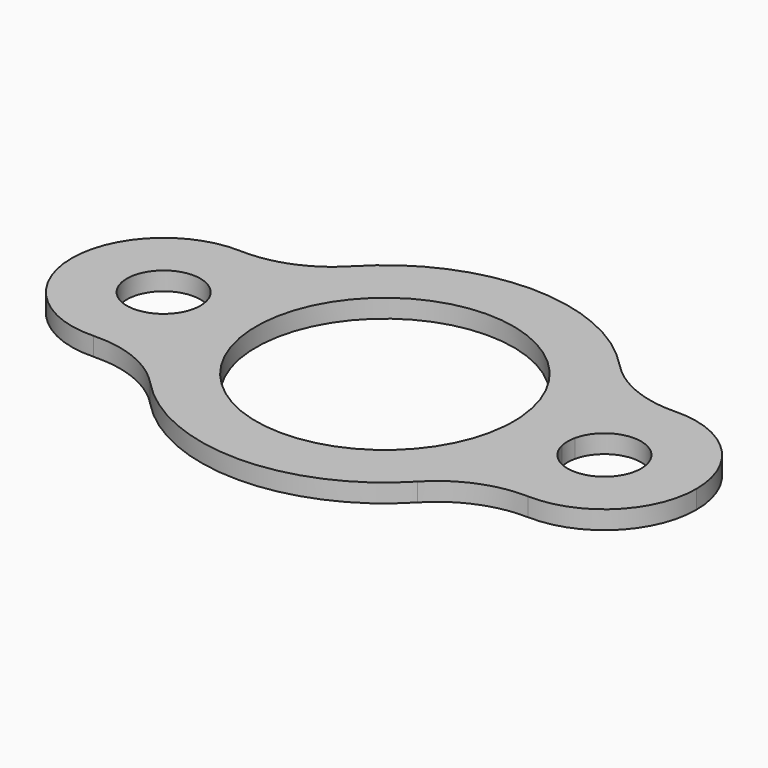
from build123d import *

# Parameters (mm, degrees)
F0_R     = 12.7
F1_DEPTH = 6.35
F2_R     = 38.1


# Not quite as in the source:
# - a length typed as a fraction of an inch, garbled in the dataset ("3 / 203.2 mm" for 3/8 in), is restored


with BuildPart() as f1:
    # F0 (on Top) → F1 (new body)
    with BuildSketch(Plane.XY):
        with BuildLine():
            ThreePointArc((44.2896283804, 3.7724419046), (44.4098889973, 1.8879245867), (44.45, 0))
            ThreePointArc((44.45, 0), (44.4098889973, -1.8879245867), (44.2896283804, -3.7724419046))
            ThreePointArc((44.2896283804, -3.7724419046), (48.6524538165, -16.4400117074), (57.8519523886, -26.1801757984))
            ThreePointArc((57.8519523886, -26.1801757983), (61.7568132692, -14.7765359551), (63.4364387448, -2.8404646402))
            ThreePointArc((63.4364387448, -2.8404646402), (63.1147165179, 0), (63.4364387448, 2.8404646402))
            ThreePointArc((63.4364387448, 2.8404646402), (61.7568132692, 14.7765359551), (57.8519523886, 26.1801757983))
            ThreePointArc((57.8519523886, 26.1801757984), (48.6524538165, 16.4400117074), (44.2896283804, 3.7724419046))
        make_face()
        with BuildLine():
            ThreePointArc((44.2896283804, -3.7724419046), (-44.45, 0), (44.2896283804, 3.7724419046))
            ThreePointArc((44.2896283804, 3.7724419046), (48.6524538165, 16.4400117074), (57.8519523886, 26.1801757984))
            ThreePointArc((57.8519523886, 26.1801757983), (-0.1747733497, 63.499759482), (-57.9951886366, 25.8613243088))
            ThreePointArc((-57.9951886366, 25.8613243088), (-48.1929456979, 14.5475718573), (-44.6640486717, 0))
            ThreePointArc((-44.6640486717, 0), (-48.1929456979, -14.5475718573), (-57.9951886366, -25.8613243088))
            ThreePointArc((-57.9951886366, -25.8613243088), (-0.1747733497, -63.499759482), (57.8519523886, -26.1801757983))
            ThreePointArc((57.8519523886, -26.1801757984), (48.6524538165, -16.4400117074), (44.2896283804, -3.7724419046))
        make_face()
        with BuildLine():
            ThreePointArc((107.5647165179, 0), (90.6090522396, 28.09252802), (57.8519523886, 26.1801757984))
            ThreePointArc((57.8519523886, 26.1801757983), (61.7568132692, 14.7765359551), (63.4364387448, 2.8404646402))
            ThreePointArc((63.4364387448, 2.8404646402), (77.244029689, 12.6193131294), (88.5147165179, 0))
            ThreePointArc((88.5147165179, 0), (77.244029689, -12.6193131294), (63.4364387448, -2.8404646402))
            ThreePointArc((63.4364387448, -2.8404646402), (61.7568132692, -14.7765359551), (57.8519523886, -26.1801757983))
            ThreePointArc((57.8519523886, -26.1801757984), (90.6090522396, -28.09252802), (107.5647165179, 0))
        make_face()
        with BuildLine():
            ThreePointArc((-44.6640486717, 0), (-48.1929456979, 14.5475718573), (-57.9951886366, 25.8613243088))
            ThreePointArc((-57.9951886366, 25.8613243088), (-63.5, 0), (-57.9951886366, -25.8613243088))
            ThreePointArc((-57.9951886366, -25.8613243088), (-48.1929456979, -14.5475718573), (-44.6640486717, 0))
        make_face()
        with BuildLine():
            ThreePointArc((-57.9951886366, -25.8613243088), (-63.5, 0), (-57.9951886366, 25.8613243088))
            ThreePointArc((-57.9951886366, 25.8613243088), (-108.1640486717, 0), (-57.9951886366, -25.8613243088))
        make_face()
        with Locations((-76.4140486717, 0)):
            Circle(F0_R, mode=Mode.SUBTRACT)
    extrude(amount=F1_DEPTH)

    # F2
    f2_edges = [f1.edges().sort_by_distance(p)[0] for p in [
        (-57.995189, 25.861324, 3.175),
        (57.851952, 26.180176, 3.175),
        (-57.995189, -25.861324, 3.175),
        (57.851952, -26.180176, 3.175),
    ]]
    fillet(f2_edges, radius=F2_R)


solid = f1.part
